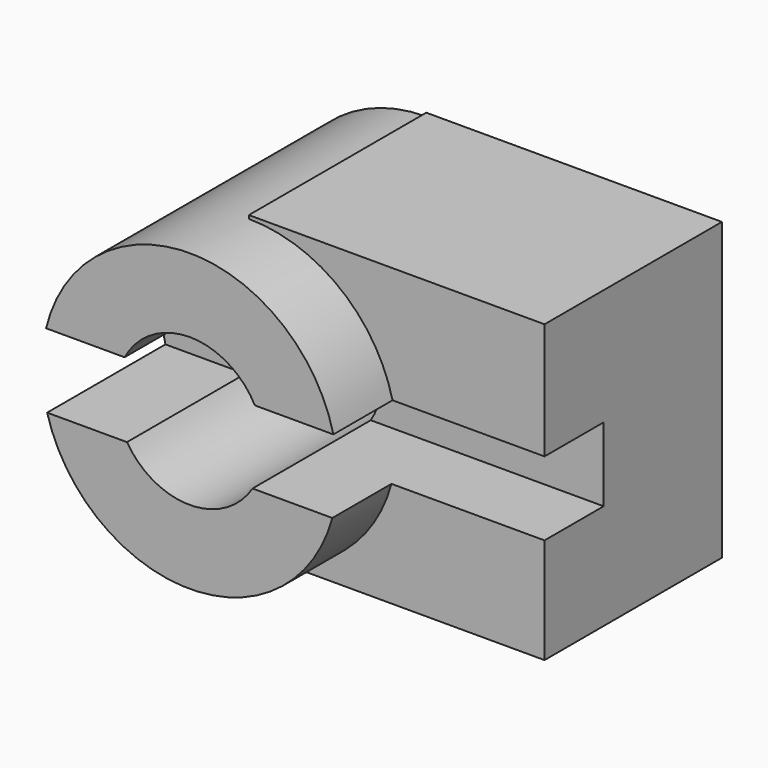
from build123d import *

# Parameters (mm, degrees)
F0_R          = 10
F0_R_2        = 5
F1_DEPTH      = 20
F2_W          = 15
F2_H          = 20
F3_DEPTH      = 20
F4_R          = 5
F5_DEPTH      = 20.001
F6_W          = 10
F6_H          = 5
F7_DEPTH      = 10.001
F7_DEPTH_BACK = 20.001


with BuildPart() as f1:
    # F0 (on Front) → F1 (new body)
    with BuildSketch(Plane.XZ):
        Circle(F0_R)
        Circle(F0_R_2, mode=Mode.SUBTRACT)
    extrude(amount=-F1_DEPTH)

    # F2 (on Right) → F3 (join)
    with BuildSketch(Plane.YZ):
        with Locations((12.5, 0.2303563431)):
            Rectangle(F2_W, F2_H)
    extrude(amount=F3_DEPTH)

    # F4 (on Front) → F5 (cut, through all)
    with BuildSketch(Plane.XZ):
        Circle(F4_R)
    extrude(amount=-F5_DEPTH, mode=Mode.SUBTRACT)

    # F6 (on Right) → F7 (cut, two sides)
    with BuildSketch(Plane.YZ) as f7_sk:
        with Locations((5, -0.1396772545)):
            Rectangle(F6_W, F6_H)
    extrude(amount=-F7_DEPTH, mode=Mode.SUBTRACT)
    extrude(f7_sk.sketch, amount=F7_DEPTH_BACK, mode=Mode.SUBTRACT)


solid = f1.part
